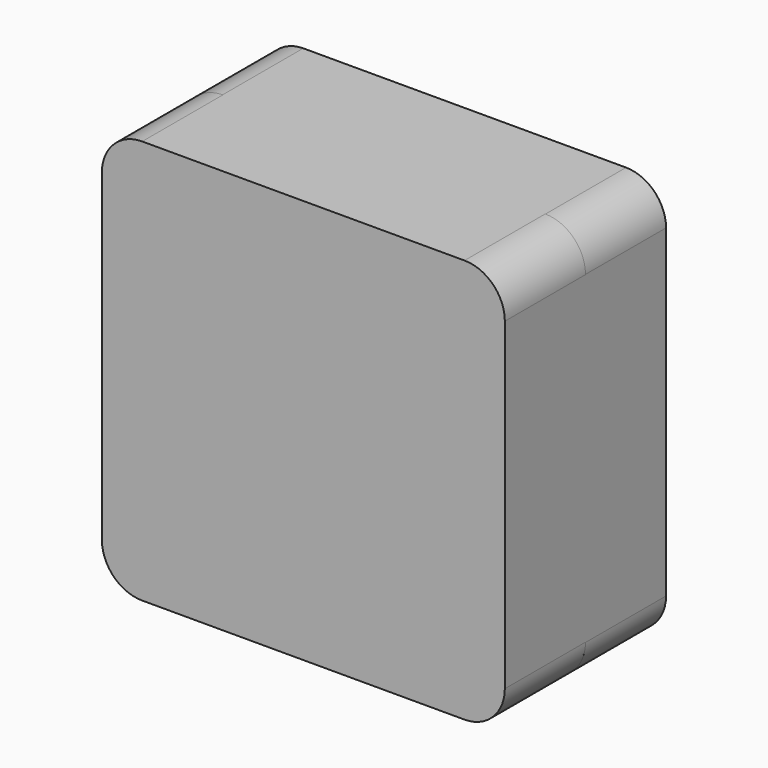
from build123d import *

# Parameters (mm, degrees)
F0_W        = 50.77206
F0_H        = 50.92827
F1_DEPTH    = 12.7
F2_R        = 5.08
F3_DEPTH    = 12.7
F4_T1_DEPTH = 38.0995000049


# Not quite as in the source:
# - a fillet or chamfer that OpenCascade refuses, or shapes differently, is made with other operations: its cross-section is extruded or revolved along the edge and cut away or added


with BuildPart() as f1:
    # F0 (on Front) → F1 (new body)
    with BuildSketch(Plane.XZ):
        Rectangle(F0_W, F0_H)
    extrude(amount=F1_DEPTH)

    # F2
    f2_edges = [f1.edges().sort_by_distance(p)[0] for p in [
        (25.38603, -6.35, 25.464135),
        (-25.38603, -6.35, 25.464135),
        (-25.38603, -6.35, -25.464135),
        (25.38603, -6.35, -25.464135),
    ]]
    fillet(f2_edges, radius=F2_R)

    # F0 (on Front) → F3 (join)
    with BuildSketch(Plane.XZ):
        Rectangle(F0_W, F0_H)
    extrude(amount=-F3_DEPTH)

    # F4: fillet of radius 5.08 on 4 edges, made by hand

    # F4_s2 → F4_t1 (cut)
    with BuildSketch(Plane.XZ.offset(-25.3997500025)):
        with BuildLine():
            ThreePointArc((-20.30613, 25.464235), (-23.8982324484, 23.9763374484), (-25.38613, 20.384235))
            Line((-25.38613, 20.384235), (-25.48773, 20.384235))
            ThreePointArc((-25.48773, 20.384235), (-25.48763, 22.924185), (-25.48763, 25.464135))
            Line((-25.48763, 25.464135), (-25.38603, 25.565735))
            ThreePointArc((-25.38603, 25.565735), (-22.84608, 25.565735), (-20.30613, 25.565835))
            Line((-20.30613, 25.565835), (-20.30613, 25.464235))
        make_face()
        with BuildLine():
            ThreePointArc((-25.38613, -20.384235), (-23.8982324484, -23.9763374484), (-20.30613, -25.464235))
            Line((-20.30613, -25.464235), (-20.30613, -25.565835))
            ThreePointArc((-20.30613, -25.565835), (-22.84608, -25.565735), (-25.38603, -25.565735))
            Line((-25.38603, -25.565735), (-25.48763, -25.464135))
            ThreePointArc((-25.48763, -25.464135), (-25.48763, -22.924185), (-25.48773, -20.384235))
            Line((-25.48773, -20.384235), (-25.38613, -20.384235))
        make_face()
        with BuildLine():
            ThreePointArc((25.38613, -20.384235), (23.8982324484, -23.9763374484), (20.30613, -25.464235))
            Line((20.30613, -25.464235), (20.30613, -25.565835))
            ThreePointArc((20.30613, -25.565835), (22.84608, -25.565735), (25.38603, -25.565735))
            Line((25.38603, -25.565735), (25.48763, -25.464135))
            ThreePointArc((25.48763, -25.464135), (25.48763, -22.924185), (25.48773, -20.384235))
            Line((25.48773, -20.384235), (25.38613, -20.384235))
        make_face()
        with BuildLine():
            ThreePointArc((20.30613, 25.464235), (23.8982324484, 23.9763374484), (25.38613, 20.384235))
            Line((25.38613, 20.384235), (25.48773, 20.384235))
            ThreePointArc((25.48773, 20.384235), (25.48763, 22.924185), (25.48763, 25.464135))
            Line((25.48763, 25.464135), (25.38603, 25.565735))
            ThreePointArc((25.38603, 25.565735), (22.84608, 25.565735), (20.30613, 25.565835))
            Line((20.30613, 25.565835), (20.30613, 25.464235))
        make_face()
    extrude(amount=F4_T1_DEPTH, mode=Mode.SUBTRACT)


solid = f1.part
